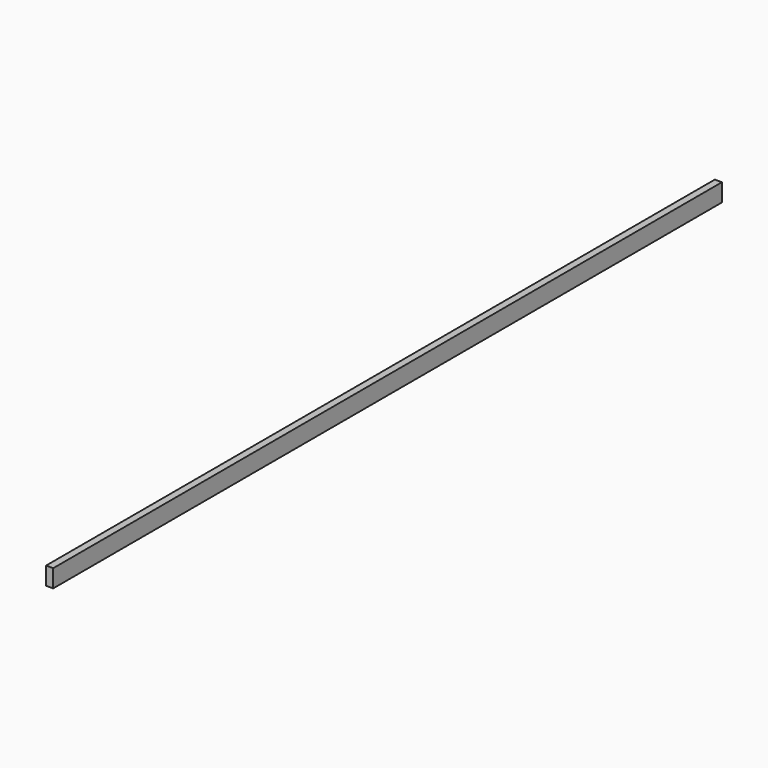
from build123d import *

# Parameters (mm, degrees)
F1_W     = 10
F1_H     = 25
F2_DEPTH = 1173


with BuildPart() as f2:
    # F1 (on Front) → F2 (new body)
    with BuildSketch(Plane.XZ):
        with Locations((5, 12.5)):
            Rectangle(F1_W, F1_H)
    extrude(amount=F2_DEPTH)


solid = f2.part
